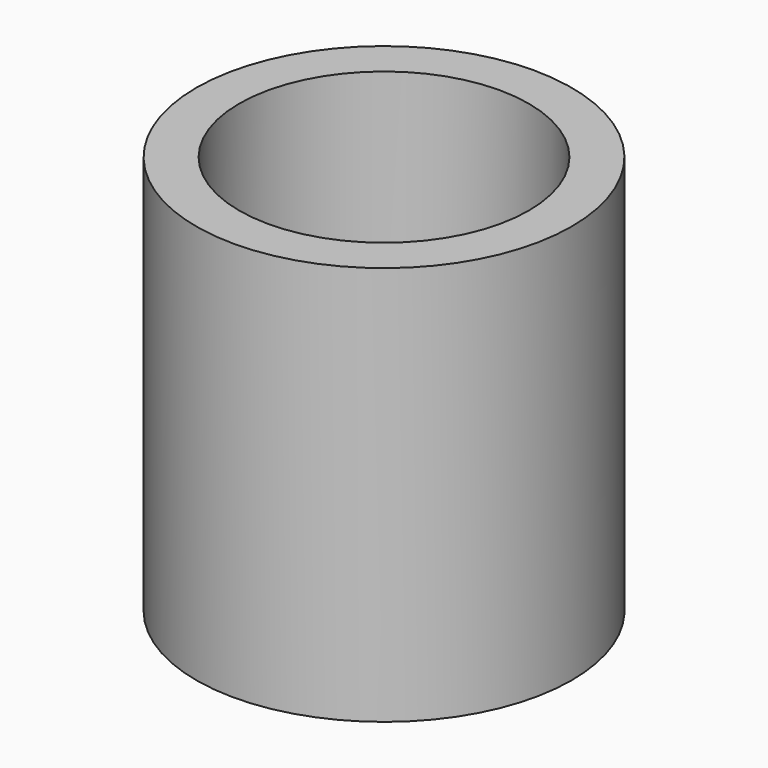
from build123d import *

# Parameters (mm, degrees)
F3_DEPTH = 25


with BuildPart() as f1:
    # F0 (on Front) → F1 (revolve)
    with BuildSketch(Plane.XZ):
        Polygon((7.25, 0), (9.4, 0), (9.4, 20), (7.25, 20), (7.25, 7), (6.25, 6), (6.25, 5), (7.25, 5), align=None)
    revolve(axis=Axis((0, 0, 5), (0, 0, 1)))

    # F2 (on Front) → F3 (cut)
    with BuildSketch(Plane.XZ):
        Polygon((5, 5), (-5, 5), (-5, 0), (0, 0), (5, 0), align=None)
    extrude(amount=-F3_DEPTH, mode=Mode.SUBTRACT)


solid = f1.part
